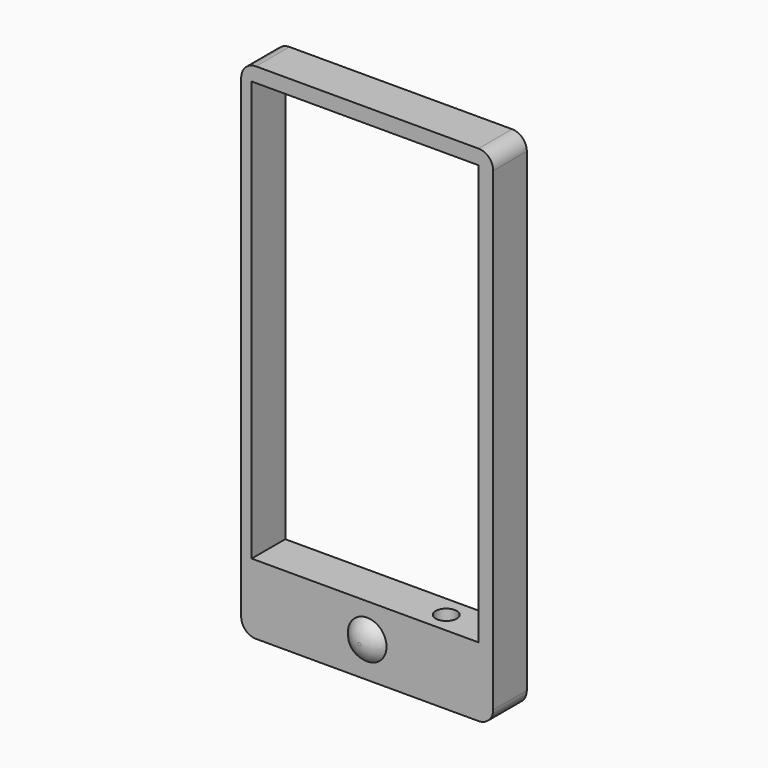
from build123d import *

# Parameters (mm, degrees)
F0_W     = 54
F0_H     = 100
F1_DEPTH = 10
F2_R     = 4.602391418
F3_DEPTH = 2.3
F6_D     = 5
F6_DEPTH = 44
F6_TIP   = 1.5021515476


# Not quite as in the source:
# - a fillet or chamfer that OpenCascade refuses, or shapes differently, is made with other operations: its cross-section is extruded or revolved along the edge and cut away or added


with BuildPart() as f1:
    # F0 (on Front) → F1 (new body)
    with BuildSketch(Plane.XZ):
        with BuildLine():
            ThreePointArc((30, 56.5), (28.9748737342, 58.9748737342), (26.5, 60))
            Line((26.5, 60), (-26.5, 60))
            ThreePointArc((-26.5, 60), (-28.9748737342, 58.9748737342), (-30, 56.5))
            Line((-30, 56.5), (-30, -56.5))
            ThreePointArc((-30, -56.5), (-28.9748737342, -58.9748737342), (-26.5, -60))
            Line((-26.5, -60), (26.5, -60))
            ThreePointArc((26.5, -60), (28.9748737342, -58.9748737342), (30, -56.5))
            Line((30, -56.5), (30, 56.5))
        make_face()
        with Locations((-0.5, 6.5)):
            Rectangle(F0_W, F0_H, mode=Mode.SUBTRACT)
    extrude(amount=F1_DEPTH)

    # F2 (on face) → F3 (join)
    with BuildSketch(Plane.XZ.offset(10)):
        with Locations((0, -51.5322610736)):
            Circle(F2_R)
    extrude(amount=F3_DEPTH)

    # F4: fillet of radius 5.069848481 on 1 edges, made by hand

    # F4_s1 → F4_t2 (revolve, cut)
    with BuildSketch(Plane.XY.offset(-51.5322610736)):
        with BuildLine():
            ThreePointArc((4.602391418, -10), (2.7706699872, -11.6880700767), (0.356063238, -12.3))
            Line((0.356063238, -12.3), (4.602391418, -12.3))
            Line((4.602391418, -12.3), (4.602391418, -10))
        make_face()
    revolve(axis=Axis((0, -12.3, -51.5322610736), (0, -1, 0)), mode=Mode.SUBTRACT)

    # F6
    with Locations(Plane(origin=(0, 0, -60), x_dir=(1, 0, 0), z_dir=(0, 0, -1))):
        with Locations((14.8790339008, 5.0806454383)):
            Hole(F6_D / 2, depth=F6_DEPTH)
            with Locations((0, 0, -(F6_DEPTH + F6_TIP / 2))):  # 118° drill point
                Cone(0, F6_D / 2, F6_TIP, mode=Mode.SUBTRACT)


solid = f1.part
